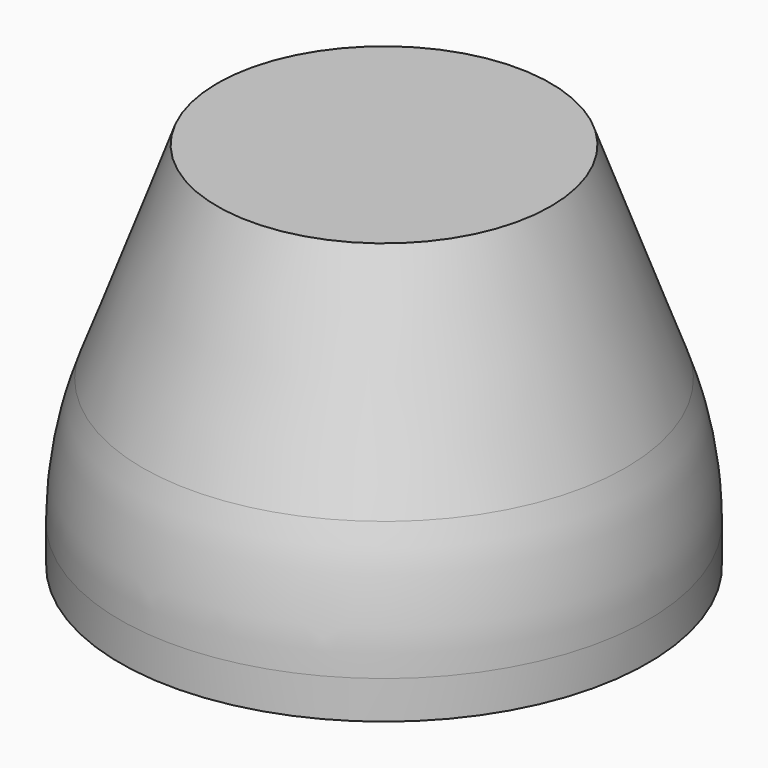
from build123d import *

# Parameters (mm, degrees)
F5_R      = 2.1
F6_DEPTH  = 30
F8_R      = 2.1
F9_DEPTH  = 30
F11_R     = 2.1
F12_DEPTH = 30
F13_R     = 1.25
F14_DEPTH = 8
F15_R     = 40


with BuildPart() as f1:
    # F0 (on Front) → F1 (revolve)
    with BuildSketch(Plane.XZ):
        Polygon((0, -2), (0, 0), (-18, 0), (-28.5, -28.8485129043), (-28.5, -40), (-22.5025773881, -40), (-15, -12), (-8, -12), (-8, -2), align=None)
    revolve(axis=Axis((0, 0, -1), (0, 0, -1)))

    # F5 (on face) → F6 (cut)
    with BuildSketch(Plane(origin=(0, -4.0048094716, -14.9461524227), x_dir=(1, 0, 0), z_dir=(0, 0.2588190451, 0.9659258263))):
        with Locations((0, -12.8830588531)):
            Circle(F5_R)
    extrude(amount=-F6_DEPTH, mode=Mode.SUBTRACT)

    # F8 (on face) → F9 (cut)
    with BuildSketch(Plane(origin=(-3.4682667397, 2.0024047358, -14.9461524227), x_dir=(0.9745560663, 0.0297636554, -0.2221589485), z_dir=(0.224143868, -0.1294095226, 0.9659258263))):
        with Locations((-11.0582542606, 6.6097063567)):
            Circle(F8_R)
    extrude(amount=-F9_DEPTH, mode=Mode.SUBTRACT)

    # F11 (on face) → F12 (cut)
    with BuildSketch(Plane(origin=(3.4682667397, 2.0024047358, -14.9461524227), x_dir=(0.9745560663, -0.0297636554, 0.2221589485), z_dir=(-0.224143868, -0.1294095226, 0.9659258263))):
        with Locations((11.0582542586, 6.6097063599)):
            Circle(F11_R)
    extrude(amount=-F12_DEPTH, mode=Mode.SUBTRACT)

    # F13 (on face) → F14 (cut)
    with BuildSketch(Plane(origin=(0, 0, -40), x_dir=(1, 0, 0), z_dir=(0, 0, -1))):
        with Locations((-22.5166604984, 13)):
            Circle(F13_R)
        with Locations((22.5166604984, 13)):
            Circle(F13_R)
        with Locations((0, -26)):
            Circle(F13_R)
    extrude(amount=-F14_DEPTH, mode=Mode.SUBTRACT)

    # F15
    f15_edges = [f1.edges().sort_by_distance(p)[0] for p in [
        (28.5, 0, -28.848513),
    ]]
    fillet(f15_edges, radius=F15_R)


solid = f1.part
